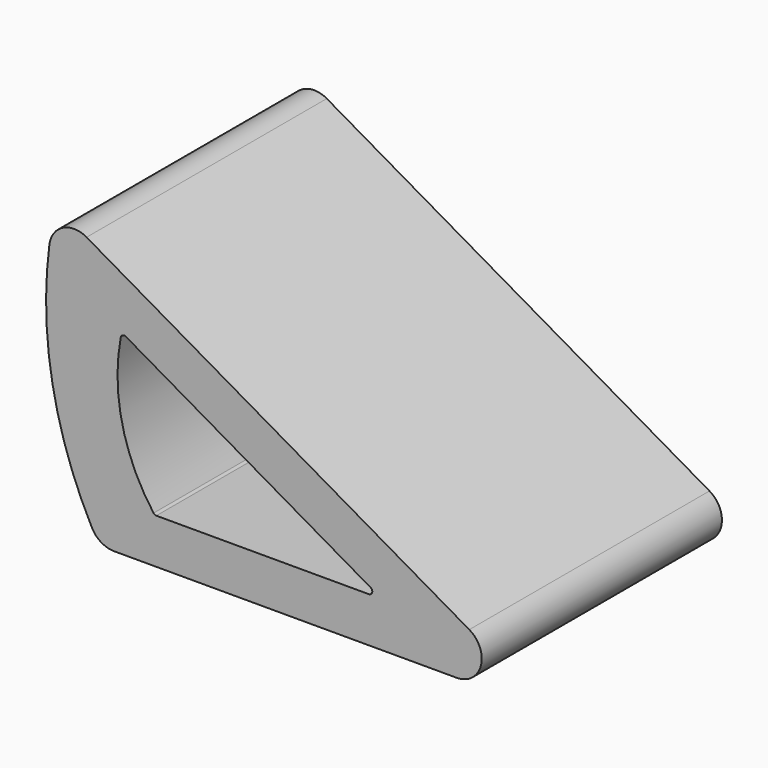
from build123d import *

# Parameters (mm, degrees)
F1_DEPTH = 20
F2_R     = 1.6600926706
F3_R     = 0.231152144


with BuildPart() as f1:
    # F0 (on Front) → F1 (new body)
    with BuildSketch(Plane.XZ):
        with BuildLine():
            ThreePointArc((-44.5080057804, 18.2982461622), (-44.856766986, 8.5238854869), (-41.6028533709, -0.6995524392))
            Line((-41.6028533709, -0.6995524392), (-11.6028533709, -0.6995524392))
            Line((-11.6028533709, -0.6995524392), (-44.5080057804, 18.2982461622))
        make_face()
        with BuildLine():
            ThreePointArc((-37.9288420081, 2.3004475608), (-40.1145449825, 7.0615839207), (-40.1195138693, 12.3004475608))
            Line((-40.1195138693, 12.3004475608), (-22.7990057936, 2.3004475608))
            Line((-22.7990057936, 2.3004475608), (-37.9288420081, 2.3004475608))
        make_face(mode=Mode.SUBTRACT)
    extrude(amount=F1_DEPTH)

    # F2
    f2_edges = [f1.edges().sort_by_distance(p)[0] for p in [
        (-11.602853, -10, -0.699552),
        (-44.508006, -10, 18.298246),
        (-41.602853, -10, -0.699552),
    ]]
    fillet(f2_edges, radius=F2_R)

    # F3
    f3_edges = [f1.edges().sort_by_distance(p)[0] for p in [
        (-22.799006, -10, 2.300448),
        (-37.928842, -10, 2.300448),
        (-40.119514, -10, 12.300448),
    ]]
    fillet(f3_edges, radius=F3_R)


solid = f1.part
